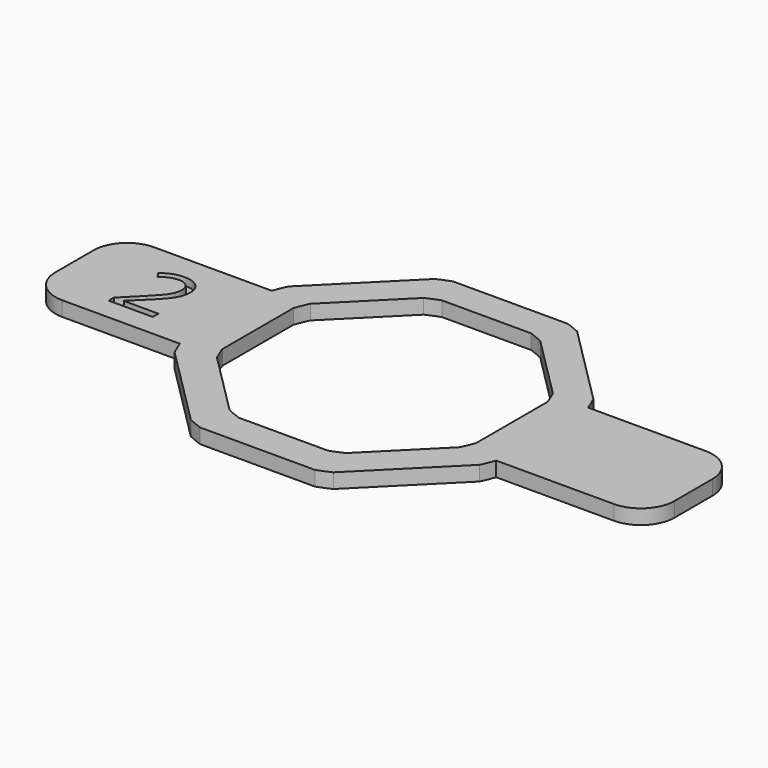
from build123d import *

# Parameters (mm, degrees)
F1_DEPTH     = 1.27
F2_DEPTH     = 1.27
F0_TEXT_SIZE = 8.1211115078
F3_DEPTH     = 0.635


# Not quite as in the source:
# - Text() gives the source's letters only with a copy of the font that has no kerning and outlines rounded to 1/6400 em; it was checked with that copy


with BuildPart() as f1:
    # F0 (on Top) → F1 (new body)
    with BuildSketch(Plane.XY):
        with BuildLine():
            Line((-6.1458364355, 13.1488852875), (-13.1488852875, 6.1458364355))
            ThreePointArc((-13.1488852875, 6.1458364355), (-13.4094515004, 5.5543766755), (-13.6434285714, 4.9519033323))
            Line((-13.6434285714, 4.9519033323), (-13.6434285714, -4.9519033323))
            ThreePointArc((-13.6434285714, -4.9519033323), (-13.4094515004, -5.5543766755), (-13.1488852875, -6.1458364355))
            Line((-13.1488852875, -6.1458364355), (-6.1458364355, -13.1488852875))
            ThreePointArc((-6.1458364355, -13.1488852875), (-5.5543766755, -13.4094515004), (-4.9519033323, -13.6434285714))
            Line((-4.9519033323, -13.6434285714), (4.9519033323, -13.6434285714))
            ThreePointArc((4.9519033323, -13.6434285714), (5.5543766755, -13.4094515004), (6.1458364355, -13.1488852875))
            Line((6.1458364355, -13.1488852875), (13.1488852875, -6.1458364355))
            ThreePointArc((13.1488852875, -6.1458364355), (13.4094515004, -5.5543766755), (13.6434285714, -4.9519033323))
            Line((13.6434285714, -4.9519033323), (13.6434285714, 4.9519033323))
            ThreePointArc((13.6434285714, 4.9519033323), (13.4094515004, 5.5543766755), (13.1488852875, 6.1458364355))
            Line((13.1488852875, 6.1458364355), (6.1458364355, 13.1488852875))
            ThreePointArc((6.1458364355, 13.1488852875), (5.5543766755, 13.4094515004), (4.9519033323, 13.6434285714))
            Line((4.9519033323, 13.6434285714), (-4.9519033323, 13.6434285714))
            ThreePointArc((-4.9519033323, 13.6434285714), (-5.5543766755, 13.4094515004), (-6.1458364355, 13.1488852875))
        make_face()
        with BuildLine():
            ThreePointArc((10.4981443223, 5.0898574374), (10.7621380976, 4.4995699253), (10.9928626115, 3.8955018339))
            Line((10.9928626115, 3.8955018339), (10.9928626115, -3.7833646641))
            ThreePointArc((10.9928626115, -3.7833646641), (10.7621380976, -4.3874327555), (10.4981443223, -4.9777202676))
            Line((10.4981443223, -4.9777202676), (5.0683657497, -10.4074988401))
            ThreePointArc((5.0683657497, -10.4074988401), (4.4780782376, -10.6714926155), (3.8740101462, -10.9022171294))
            Line((3.8740101462, -10.9022171294), (-3.8048563517, -10.9022171294))
            ThreePointArc((-3.8048563517, -10.9022171294), (-4.4089244431, -10.6714926155), (-4.9992119552, -10.4074988401))
            Line((-4.9992119552, -10.4074988401), (-10.4289905278, -4.9777202676))
            ThreePointArc((-10.4289905278, -4.9777202676), (-10.6929843031, -4.3874327555), (-10.923708817, -3.7833646641))
            Line((-10.923708817, -3.7833646641), (-10.923708817, 3.8955018339))
            ThreePointArc((-10.923708817, 3.8955018339), (-10.6929843031, 4.4995699253), (-10.4289905278, 5.0898574374))
            Line((-10.4289905278, 5.0898574374), (-4.9992119552, 10.5196360099))
            ThreePointArc((-4.9992119552, 10.5196360099), (-4.4089244431, 10.7836297852), (-3.8048563517, 11.0143542992))
            Line((-3.8048563517, 11.0143542992), (3.8740101462, 11.0143542992))
            ThreePointArc((3.8740101462, 11.0143542992), (4.4780782376, 10.7836297852), (5.0683657497, 10.5196360099))
            Line((5.0683657497, 10.5196360099), (10.4981443223, 5.0898574374))
        make_face(mode=Mode.SUBTRACT)
    extrude(amount=F1_DEPTH)

    # F0 (on Top) → F2 (join)
    with BuildSketch(Plane.XY):
        with BuildLine():
            Line((-13.6434285714, -4.9519033323), (-13.6434285714, 4.9519033323))
            Line((-13.6434285714, 4.9519033323), (-23.8034285714, 4.9519033323))
            ThreePointArc((-23.8034285714, 4.9519033323), (-25.856058542, 4.10167616), (-26.7062857143, 2.0490461894))
            Line((-26.7062857143, 2.0490461894), (-26.7062857143, -2.0490461894))
            ThreePointArc((-26.7062857143, -2.0490461894), (-25.856058542, -4.10167616), (-23.8034285714, -4.9519033323))
            Line((-23.8034285714, -4.9519033323), (-13.6434285714, -4.9519033323))
        make_face()
        with BuildLine():
            Line((-17.514245467, -2.433897436), (-17.514245467, -3.0442497227))
            Line((-17.514245467, -3.0442497227), (-21.3248232573, -3.0442497227))
            Line((-21.3248232573, -3.0442497227), (-21.3248232573, -2.4770408409))
            Line((-21.3248232573, -2.4770408409), (-19.7983080786, -0.9429121201))
            add(Edge.make_bspline(
                [(-19.7983080786, -0.9429121201), (-19.1004000584, -0.2361216342), (-18.8783384156, 0.0652477382)],
                knots=[0, 0, 0, 1, 1, 1], degree=2))
            add(Edge.make_bspline(
                [(-18.8783384156, 0.0652477382), (-18.6562767728, 0.3666171106), (-18.5452459514, 0.652124937)],
                knots=[0, 0, 0, 1, 1, 1], degree=2))
            add(Edge.make_bspline(
                [(-18.5452459514, 0.652124937), (-18.43421513, 0.9376327635), (-18.43421513, 1.2662839948)],
                knots=[0, 0, 0, 1, 1, 1], degree=2))
            add(Edge.make_bspline(
                [(-18.43421513, 1.2662839948), (-18.43421513, 1.7307100591), (-18.7159161854, 2.0022597252)],
                knots=[0, 0, 0, 1, 1, 1], degree=2))
            add(Edge.make_bspline(
                [(-18.7159161854, 2.0022597252), (-18.9976172408, 2.2738093912), (-19.497573168, 2.2738093912)],
                knots=[0, 0, 0, 1, 1, 1], degree=2))
            add(Edge.make_bspline(
                [(-19.497573168, 2.2738093912), (-19.8579474912, 2.2738093912), (-20.1815230278, 2.154530566)],
                knots=[0, 0, 0, 1, 1, 1], degree=2))
            add(Edge.make_bspline(
                [(-20.1815230278, 2.154530566), (-20.5050985645, 2.0352517407), (-20.9010027505, 1.7218275934)],
                knots=[0, 0, 0, 1, 1, 1], degree=2))
            Line((-20.9010027505, 1.7218275934), (-21.2499567606, 2.16975765))
            add(Edge.make_bspline(
                [(-21.2499567606, 2.16975765), (-20.4492659229, 2.8359425784), (-19.5051867101, 2.8359425784)],
                knots=[0, 0, 0, 1, 1, 1], degree=2))
            add(Edge.make_bspline(
                [(-19.5051867101, 2.8359425784), (-18.6879998646, 2.8359425784), (-18.2242082621, 2.4178322281)],
                knots=[0, 0, 0, 1, 1, 1], degree=2))
            add(Edge.make_bspline(
                [(-18.2242082621, 2.4178322281), (-17.7604166596, 1.9997218778), (-17.7604166596, 1.2942003156)],
                knots=[0, 0, 0, 1, 1, 1], degree=2))
            add(Edge.make_bspline(
                [(-17.7604166596, 1.2942003156), (-17.7604166596, 0.7422185178), (-18.0700340358, 0.2029259567)],
                knots=[0, 0, 0, 1, 1, 1], degree=2))
            add(Edge.make_bspline(
                [(-18.0700340358, 0.2029259567), (-18.379651412, -0.3363666043), (-19.2272924257, -1.1611669919)],
                knots=[0, 0, 0, 1, 1, 1], degree=2))
            Line((-19.2272924257, -1.1611669919), (-20.4962160988, -2.4021743441))
            Line((-20.4962160988, -2.4021743441), (-20.4962160988, -2.433897436))
            Line((-20.4962160988, -2.433897436), (-17.514245467, -2.433897436))
        make_face(mode=Mode.SUBTRACT)
        with BuildLine():
            Line((23.8034285714, 4.9519033323), (13.6434285714, 4.9519033323))
            Line((13.6434285714, 4.9519033323), (13.6434285714, -4.9519033323))
            Line((13.6434285714, -4.9519033323), (23.8034285714, -4.9519033323))
            ThreePointArc((23.8034285714, -4.9519033323), (25.856058542, -4.10167616), (26.7062857143, -2.0490461894))
            Line((26.7062857143, -2.0490461894), (26.7062857143, 2.0490461894))
            ThreePointArc((26.7062857143, 2.0490461894), (25.856058542, 4.10167616), (23.8034285714, 4.9519033323))
        make_face()
    extrude(amount=F2_DEPTH)

    # F0 (on Top) → F3 (join)
    with BuildSketch(Plane.XY):
        with Locations((-21.721996367, -3.0442497227)):
            Text('2', F0_TEXT_SIZE, font='Open Sans', text_align=(TextAlign.LEFT, TextAlign.BOTTOM))
    extrude(amount=F3_DEPTH)


solid = f1.part
